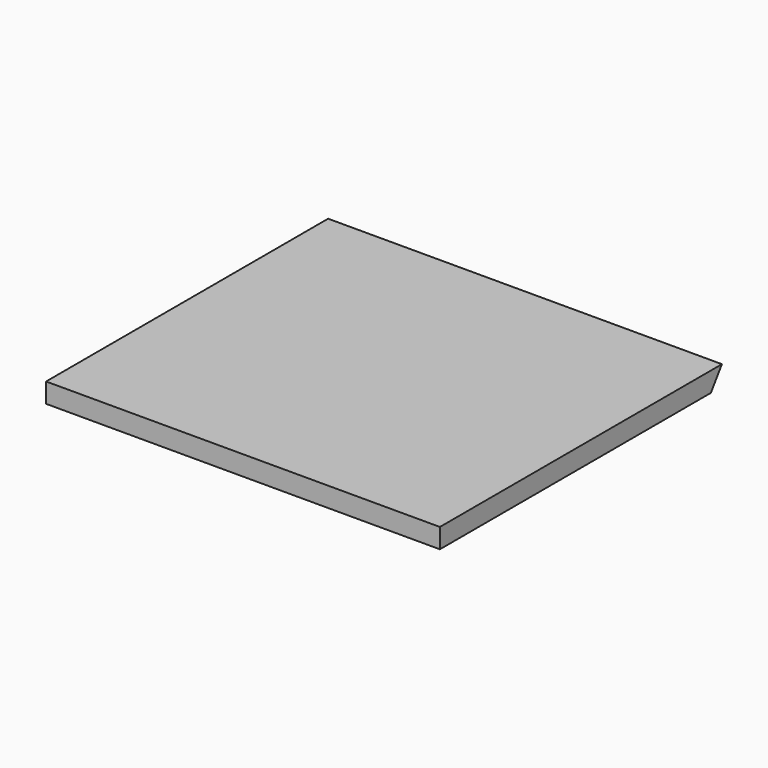
from build123d import *

# Parameters (mm, degrees)
F0_W        = 100
F0_H        = 91.02
F1_DEPTH    = 2.5
F2_T1_DEPTH = 136.8826681999


# Not quite as in the source:
# - a fillet or chamfer that OpenCascade refuses, or shapes differently, is made with other operations: its cross-section is extruded or revolved along the edge and cut away or added


with BuildPart() as f1:
    # F0 (on Top) → F1 (new body, symmetric)
    with BuildSketch(Plane.XY):
        with Locations((-50, 45.51)):
            Rectangle(F0_W, F0_H)
    extrude(amount=F1_DEPTH, both=True)

    # F2: chamfer of 5 x 7.1407400337 on 1 edges, made by hand

    # F2_s2 → F2_t1 (cut)
    with BuildSketch(Plane.YZ.offset(-118.4413340999)):
        Polygon((91.02, 4.6407400337), (86.02, -2.5), (91.02, -2.5), align=None)
    extrude(amount=F2_T1_DEPTH, mode=Mode.SUBTRACT)


solid = f1.part
